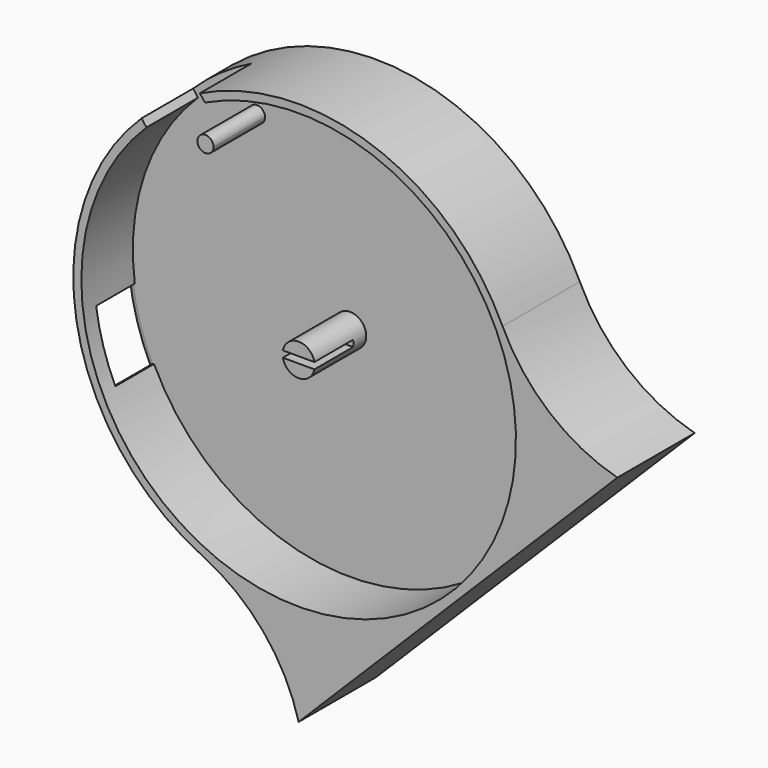
from build123d import *

# Parameters (mm, degrees)
F0_R          = 88.9
F1_DEPTH      = 12.7
F2_R          = 88.9
F2_R_2        = 82.55
F2_R_3        = 6.35
F3_DEPTH      = 25.4
F5_DEPTH      = 25.4
F7_DEPTH      = 25.4
F8_W          = 12.7
F8_H          = 1.27
F9_DEPTH      = 19.05
F10_W         = 19.05
F10_H         = 25.4
F11_DEPTH     = 88.901
F12_T1_DEPTH  = 19.05
F12_T6_ANGLE  = 25.274429264
F12_T12_ANGLE = 25.274429264
F12_T19_ANGLE = 25.274429264
F12_T23_DEPTH = 24.7827133537
F12_T30_ANGLE = 25.274429264
F12_T34_DEPTH = 24.7827133537
F12_T41_DEPTH = 29.3229812516
F12_T45_ANGLE = 25.274429264
F12_T52_ANGLE = 25.274429264
F12_T56_DEPTH = 29.3229812516
F14_DEPTH     = 25.4
F16_DEPTH     = 38.1
F20_DEPTH     = 25.4


# Not quite as in the source:
# - a fillet or chamfer that OpenCascade refuses, or shapes differently, is made with other operations: its cross-section is extruded or revolved along the edge and cut away or added


with BuildPart() as f1:
    # F0 (on Front) → F1 (new body)
    with BuildSketch(Plane.XZ):
        Circle(F0_R)
    extrude(amount=F1_DEPTH)

    # F2 (on face) → F3 (join)
    with BuildSketch(Plane.XZ.offset(12.7)):
        Circle(F2_R)
        Circle(F2_R_2, mode=Mode.SUBTRACT)
        Circle(F2_R_3)
    extrude(amount=F3_DEPTH)

    # F4 (on face) → F5 (cut)
    with BuildSketch(Plane.XZ.offset(38.1)):
        with BuildLine():
            Line((-34.9300524425, 74.7956812681), (-38.9724939218, 79.9021571518))
            ThreePointArc((-38.9724939218, 79.9021571518), (-51.1040456605, 72.7432919047), (-61.9525410202, 63.7580791833))
            Line((-61.9525410202, 63.7580791833), (-58.1372414147, 58.6051504621))
            ThreePointArc((-58.1372414147, 58.6051504621), (-47.2325482948, 67.7022073612), (-34.9300524425, 74.7956812681))
        make_face()
    extrude(amount=-F5_DEPTH, mode=Mode.SUBTRACT)

    # F6 (on face) → F7 (join)
    with BuildSketch(Plane.XZ.offset(12.7)):
        with BuildLine():
            ThreePointArc((-33.5668462981, 63.0071964846), (-35.8100364522, 66.042382708), (-39.3699048248, 64.7887501268))
            Line((-39.3699048248, 64.7887501268), (-34.1137877714, 61.2256428423))
            ThreePointArc((-34.1137877714, 61.2256428423), (-33.7066600747, 62.0753866387), (-33.5668462981, 63.0071964846))
        make_face()
        with BuildLine():
            Line((-34.1137877714, 61.2256428423), (-39.3699048248, 64.7887501268))
            ThreePointArc((-39.3699048248, 64.7887501268), (-38.5233999404, 60.3791379579), (-34.1137877714, 61.2256428423))
        make_face()
    extrude(amount=F7_DEPTH)

    # F8 (on face) → F9 (cut)
    with BuildSketch(Plane.XZ.offset(38.1)):
        with Locations((0, 0.635)):
            Rectangle(F8_W, F8_H)
        with Locations((0, -0.635)):
            Rectangle(F8_W, F8_H)
    extrude(amount=-F9_DEPTH, mode=Mode.SUBTRACT)

    # F10 (on Right) → F11 (cut, through all)
    with BuildSketch(Plane.YZ):
        with Locations((-22.225, -24.1626900017)):
            Rectangle(F10_W, F10_H)
    extrude(amount=-F11_DEPTH, mode=Mode.SUBTRACT)

    # F12: fillet of radius 2.54 on 4 edges, made by hand

    # F12_s2 → F12_t1 (cut)
    with BuildSketch(Plane.XZ.offset(12.7)):
        with BuildLine():
            ThreePointArc((-88.4242248071, -9.1851220606), (-87.5985568369, -10.8092447226), (-85.897818384, -11.4626900017))
            Line((-85.897818384, -11.4626900017), (-88.1579079716, -11.4626900017))
            ThreePointArc((-88.1579079716, -11.4626900017), (-88.2984101391, -10.3247647385), (-88.4242248071, -9.1851220606))
        make_face()
        with BuildLine():
            ThreePointArc((-79.1073144645, -40.5615926488), (-79.0145016969, -38.078305753), (-76.8471054798, -36.8626900017))
            Line((-76.8471054798, -36.8626900017), (-80.8971698259, -36.8626900017))
            ThreePointArc((-80.8971698259, -36.8626900017), (-80.0236166295, -38.7224841861), (-79.1073144645, -40.5615926488))
        make_face()
    extrude(amount=F12_T1_DEPTH, mode=Mode.SUBTRACT)


with BuildPart() as f12_tool4:
    # F12_s5 → F12_t6 (revolve)
    with BuildSketch(Plane(origin=(0, 0, 0), x_dir=(0, 1, 0), z_dir=(0.478540272, 0, -0.8780656058))):
        with BuildLine():
            ThreePointArc((-10.16, -88.9), (-11.9560512242, -88.1560512242), (-12.7, -86.36))
            Line((-12.7, -86.36), (-12.7, -88.9))
            Line((-12.7, -88.9), (-10.16, -88.9))
        make_face()
    revolve(axis=Axis((0, -12.7, 0), (0, 1, 0)), revolution_arc=F12_T6_ANGLE)

    split(bisect_by=Plane.XY.offset(-11.4626900017), keep=Keep.BOTTOM)

    split(bisect_by=Plane.XY.offset(-36.8626900017), keep=Keep.TOP)


with BuildPart() as f1_1:
    add(f1.part)

    # F12_t3: cut F12_tool4
    add(f12_tool4.part, mode=Mode.SUBTRACT)


with BuildPart() as f12_tool10:
    # F12_s11 → F12_t12 (revolve)
    with BuildSketch(Plane(origin=(0, 0, 0), x_dir=(0, 1, 0), z_dir=(0.478540272, 0, -0.8780656058))):
        with BuildLine():
            ThreePointArc((-34.29, -88.9), (-32.4939487758, -88.1560512242), (-31.75, -86.36))
            Line((-31.75, -86.36), (-31.75, -88.9))
            Line((-31.75, -88.9), (-34.29, -88.9))
        make_face()
    revolve(axis=Axis((0, -31.75, 0), (0, 1, 0)), revolution_arc=F12_T12_ANGLE)

    split(bisect_by=Plane.XY.offset(-36.8626900017), keep=Keep.TOP)

    split(bisect_by=Plane.XY.offset(-11.4626900017), keep=Keep.BOTTOM)


with BuildPart() as f1_2:
    add(f1_1.part)

    # F12_t9: cut F12_tool10
    add(f12_tool10.part, mode=Mode.SUBTRACT)


with BuildPart() as f12_tool17:
    # F12_s18 → F12_t19 (revolve)
    with BuildSketch(Plane(origin=(0, 0, 0), x_dir=(0, 1, 0), z_dir=(0.478540272, 0, -0.8780656058))):
        with BuildLine():
            ThreePointArc((-34.29, -88.9), (-32.4939487758, -88.1560512242), (-31.75, -86.36))
            Line((-31.75, -86.36), (-31.75, -88.9))
            Line((-31.75, -88.9), (-34.29, -88.9))
        make_face()
    revolve(axis=Axis((0, -31.75, 0), (0, 1, 0)), revolution_arc=F12_T19_ANGLE)

    split(bisect_by=Plane.XY.offset(-11.4626900017), keep=Keep.TOP)


with BuildPart() as f12_tool21:
    # F12_s22 → F12_t23 (new body)
    with BuildSketch(Plane.XZ.offset(37.4827133537)):
        with BuildLine():
            ThreePointArc((-88.4242248071, -9.1851220606), (-87.5985568369, -10.8092447226), (-85.897818384, -11.4626900017))
            Line((-85.897818384, -11.4626900017), (-88.1579079716, -11.4626900017))
            ThreePointArc((-88.1579079716, -11.4626900017), (-88.2984101391, -10.3247647385), (-88.4242248071, -9.1851220606))
        make_face()
    extrude(amount=-F12_T23_DEPTH)

    split(bisect_by=Plane.XZ.offset(31.75), keep=Keep.TOP)


with BuildPart() as f12_tool17_1:
    add(f12_tool17.part)

    # F12_t25: intersect F12_tool21
    add(f12_tool21.part, mode=Mode.INTERSECT)


with BuildPart() as f1_3:
    add(f1_2.part)

    # F12_t15: cut F12_tool17
    add(f12_tool17_1.part, mode=Mode.SUBTRACT)


with BuildPart() as f12_tool28:
    # F12_s29 → F12_t30 (revolve)
    with BuildSketch(Plane(origin=(0, 0, 0), x_dir=(0, 1, 0), z_dir=(0.478540272, 0, -0.8780656058))):
        with BuildLine():
            ThreePointArc((-10.16, -88.9), (-11.9560512242, -88.1560512242), (-12.7, -86.36))
            Line((-12.7, -86.36), (-12.7, -88.9))
            Line((-12.7, -88.9), (-10.16, -88.9))
        make_face()
    revolve(axis=Axis((0, -12.7, 0), (0, 1, 0)), revolution_arc=F12_T30_ANGLE)

    split(bisect_by=Plane.XY.offset(-11.4626900017), keep=Keep.TOP)


with BuildPart() as f12_tool32:
    # F12_s33 → F12_t34 (new body)
    with BuildSketch(Plane.XZ.offset(31.75)):
        with BuildLine():
            ThreePointArc((-88.4242248071, -9.1851220606), (-87.5985568369, -10.8092447226), (-85.897818384, -11.4626900017))
            Line((-85.897818384, -11.4626900017), (-88.1579079716, -11.4626900017))
            ThreePointArc((-88.1579079716, -11.4626900017), (-88.2984101391, -10.3247647385), (-88.4242248071, -9.1851220606))
        make_face()
    extrude(amount=-F12_T34_DEPTH)

    split(bisect_by=Plane.XZ.offset(12.7), keep=Keep.BOTTOM)


with BuildPart() as f12_tool28_1:
    add(f12_tool28.part)

    # F12_t36: intersect F12_tool32
    add(f12_tool32.part, mode=Mode.INTERSECT)


with BuildPart() as f1_4:
    add(f1_3.part)

    # F12_t26: cut F12_tool28
    add(f12_tool28_1.part, mode=Mode.SUBTRACT)


with BuildPart() as f12_tool39:
    # F12_s40 → F12_t41 (new body)
    with BuildSketch(Plane.XZ.offset(31.75)):
        with BuildLine():
            ThreePointArc((-79.1073144645, -40.5615926488), (-79.0145016969, -38.078305753), (-76.8471054798, -36.8626900017))
            Line((-76.8471054798, -36.8626900017), (-80.8971698259, -36.8626900017))
            ThreePointArc((-80.8971698259, -36.8626900017), (-80.0236166295, -38.7224841861), (-79.1073144645, -40.5615926488))
        make_face()
    extrude(amount=-F12_T41_DEPTH)

    split(bisect_by=Plane.XZ.offset(12.7), keep=Keep.BOTTOM)


with BuildPart() as f12_tool43:
    # F12_s44 → F12_t45 (revolve)
    with BuildSketch(Plane(origin=(0, 0, 0), x_dir=(0, 1, 0), z_dir=(0.478540272, 0, -0.8780656058))):
        with BuildLine():
            ThreePointArc((-10.16, -88.9), (-11.9560512242, -88.1560512242), (-12.7, -86.36))
            Line((-12.7, -86.36), (-12.7, -88.9))
            Line((-12.7, -88.9), (-10.16, -88.9))
        make_face()
    revolve(axis=Axis((0, -12.7, 0), (0, 1, 0)), revolution_arc=F12_T45_ANGLE)

    split(bisect_by=Plane.XY.offset(-36.8626900017), keep=Keep.BOTTOM)


with BuildPart() as f12_tool39_1:
    add(f12_tool39.part)

    # F12_t47: intersect F12_tool43
    add(f12_tool43.part, mode=Mode.INTERSECT)


with BuildPart() as f1_5:
    add(f1_4.part)

    # F12_t37: cut F12_tool39
    add(f12_tool39_1.part, mode=Mode.SUBTRACT)


with BuildPart() as f12_tool50:
    # F12_s51 → F12_t52 (revolve)
    with BuildSketch(Plane(origin=(0, 0, 0), x_dir=(0, 1, 0), z_dir=(0.478540272, 0, -0.8780656058))):
        with BuildLine():
            ThreePointArc((-34.29, -88.9), (-32.4939487758, -88.1560512242), (-31.75, -86.36))
            Line((-31.75, -86.36), (-31.75, -88.9))
            Line((-31.75, -88.9), (-34.29, -88.9))
        make_face()
    revolve(axis=Axis((0, -31.75, 0), (0, 1, 0)), revolution_arc=F12_T52_ANGLE)

    split(bisect_by=Plane.XY.offset(-36.8626900017), keep=Keep.BOTTOM)


with BuildPart() as f12_tool54:
    # F12_s55 → F12_t56 (new body)
    with BuildSketch(Plane.XZ.offset(42.0229812516)):
        with BuildLine():
            ThreePointArc((-79.1073144645, -40.5615926488), (-79.0145016969, -38.078305753), (-76.8471054798, -36.8626900017))
            Line((-76.8471054798, -36.8626900017), (-80.8971698259, -36.8626900017))
            ThreePointArc((-80.8971698259, -36.8626900017), (-80.0236166295, -38.7224841861), (-79.1073144645, -40.5615926488))
        make_face()
    extrude(amount=-F12_T56_DEPTH)

    split(bisect_by=Plane.XZ.offset(31.75), keep=Keep.TOP)


with BuildPart() as f12_tool50_1:
    add(f12_tool50.part)

    # F12_t58: intersect F12_tool54
    add(f12_tool54.part, mode=Mode.INTERSECT)


with BuildPart() as f1_6:
    add(f1_5.part)

    # F12_t48: cut F12_tool50
    add(f12_tool50_1.part, mode=Mode.SUBTRACT)

    # F13 (on face) → F14 (cut)
    with BuildSketch(Plane.XZ.offset(38.1)):
        with BuildLine():
            ThreePointArc((-34.9300524425, 74.7956812681), (44.3341102926, 69.6346836323), (82.55, 0))
            ThreePointArc((82.55, 0), (-31.7432923719, -76.2027944986), (-58.1372414147, 58.6051504621))
            Line((-58.1372414147, 58.6051504621), (-60.0455804339, 61.1825456757))
            ThreePointArc((-60.0455804339, 61.1825456757), (-33.1765598149, -79.0448701931), (85.725, 0))
            ThreePointArc((85.725, 0), (45.721772873, 72.5141028376), (-36.9532177975, 77.3513756788))
            Line((-36.9532177975, 77.3513756788), (-34.9300524425, 74.7956812681))
        make_face()
    extrude(amount=-F14_DEPTH, mode=Mode.SUBTRACT)

    # F15 (on face) → F16 (join)
    with BuildSketch(Plane(origin=(0, 0, 0), x_dir=(-1, 0, 0), z_dir=(0, 1, 0))):
        with BuildLine():
            Line((-125.723585695, 0), (-62.8617928475, -62.8617928475))
            ThreePointArc((-62.8617928475, -62.8617928475), (-87.5758152323, -15.286810864), (-80.4411250184, 37.8475283972))
            ThreePointArc((-80.4411250184, 37.8475283972), (-98.9019872856, 13.9221865314), (-125.723585695, 0))
        make_face()
        with BuildLine():
            ThreePointArc((37.8475283972, -80.4411250184), (19.3906418907, -86.7595124875), (0, -88.9))
            ThreePointArc((0, -88.9), (-34.0205571373, -82.1328904403), (-62.8617928475, -62.8617928475))
            Line((-62.8617928475, -62.8617928475), (0, -125.723585695))
            ThreePointArc((0, -125.723585695), (13.9221865314, -98.9019872856), (37.8475283972, -80.4411250184))
        make_face()
    extrude(amount=-F16_DEPTH)

    # F19 (on face) → F20 (cut)
    with BuildSketch(Plane(origin=(-61.6045569905, 0, 61.6045569905), x_dir=(0, -1, 0), z_dir=(-0.7071067812, 0, 0.7071067812))):
        Polygon((25.1616425812, -3.5754330456), (17.159935087, -3.5754330456), (17.159935087, -10.567618534), (11.9749652222, -10.567618534), (21.1607888341, -15.9158930182), (30.4591618478, -10.567618534), (25.1616425812, -10.567618534), align=None)
    extrude(amount=F20_DEPTH, mode=Mode.SUBTRACT)


solid = f1_6.part
